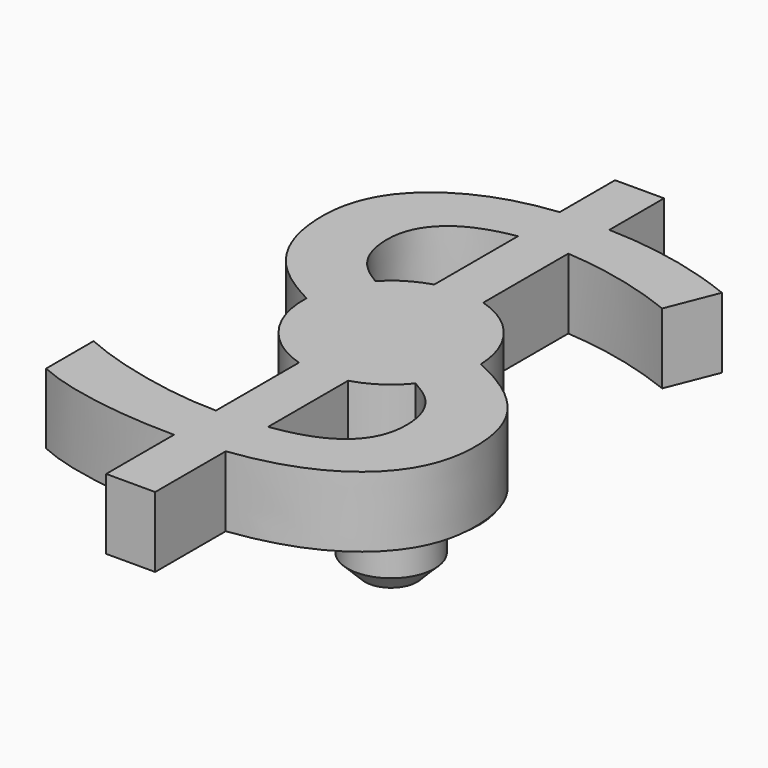
from build123d import *

# Parameters (mm, degrees)
F0_TEXT_SIZE = 44.2557812979
F1_DEPTH     = 4
F2_R         = 5
F3_DEPTH     = 4
F4_R         = 2.475
F5_DEPTH     = 4
F6_SIZE      = 1


# Not quite as in the source:
# - Text() gives the source's letters only with a copy of the font that has no kerning and outlines rounded to 1/6400 em; it was checked with that copy


with BuildPart() as f1:
    # F0 (on Top) → F1 (new body)
    with BuildSketch(Plane.XY):
        with Locations((-12.6301850845, -15.9320812672)):
            Text('$', F0_TEXT_SIZE, font='Open Sans', text_align=(TextAlign.LEFT, TextAlign.BOTTOM))
    extrude(amount=-F1_DEPTH)

    # F2 (on face) → F3 (join, symmetric)
    with BuildSketch(Plane(origin=(0, 0, -4), x_dir=(1, 0, 0), z_dir=(0, 0, -1))):
        Circle(F2_R)
    extrude(amount=F3_DEPTH, both=True)

    # F4 (on face) → F5 (join)
    with BuildSketch(Plane(origin=(0, 0, -8), x_dir=(1, 0, 0), z_dir=(0, 0, -1))):
        Circle(F4_R)
    extrude(amount=F5_DEPTH)

    # F6
    f6_edges = [f1.edges().sort_by_distance(p)[0] for p in [
        (-2.475, 0, -12),
    ]]
    chamfer(f6_edges, length=F6_SIZE)


solid = f1.part
